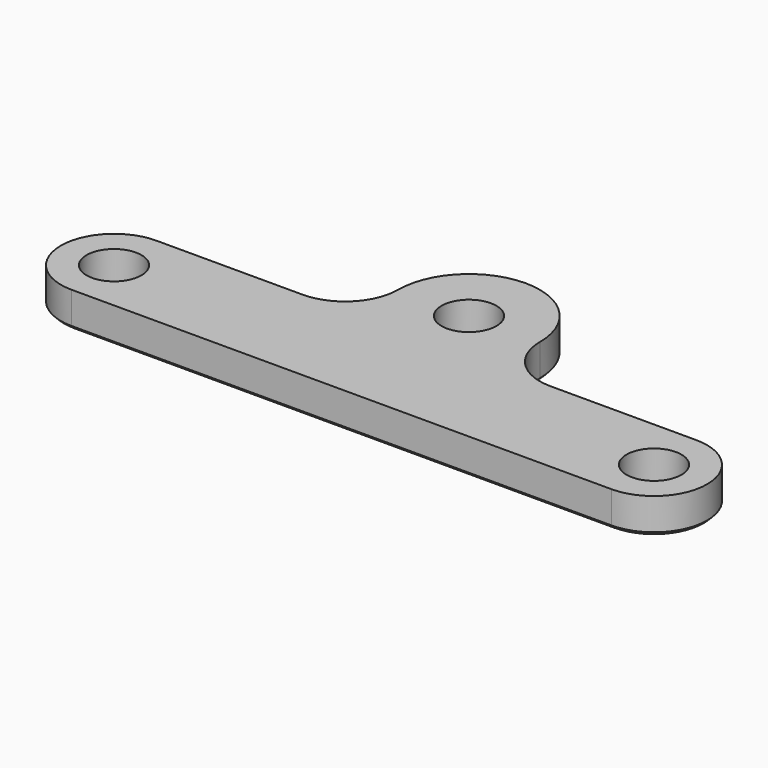
from build123d import *

# Parameters (mm, degrees)
F0_R     = 1.55
F1_DEPTH = 2
F2_R     = 2.99999
F3_SIZE  = 0.2


# Not quite as in the source:
# - a fillet or chamfer is up to 0.001 mm smaller than in the source, because OpenCascade refuses the exact size


with BuildPart() as f1:
    # F0 (on Top) → F1 (new body)
    with BuildSketch(Plane.XY):
        with BuildLine():
            ThreePointArc((-15.25, 3), (-18.25, 0), (-15.25, -3))
            Line((-15.25, -3), (15.25, -3))
            ThreePointArc((15.25, -3), (18.25, 0), (15.25, 3))
            Line((15.25, 3), (4, 3))
            Line((4, 3), (-4, 3))
            Line((-4, 3), (-15.25, 3))
        make_face()
        with Locations((-15.25, 0)):
            Circle(F0_R, mode=Mode.SUBTRACT)
        with Locations((15.25, 0)):
            Circle(F0_R, mode=Mode.SUBTRACT)
        with BuildLine():
            Line((-4, 6), (-4, 3))
            Line((-4, 3), (4, 3))
            Line((4, 3), (4, 6))
            ThreePointArc((4, 6), (0, 10), (-4, 6))
        make_face()
        with Locations((0, 6)):
            Circle(F0_R, mode=Mode.SUBTRACT)
    extrude(amount=F1_DEPTH)

    # F2 (radius 3 in the source; OpenCascade refuses exactly that, so slightly less here)
    f2_edges = [f1.edges().sort_by_distance(p)[0] for p in [
        (4, 3, 1),
        (-4, 3, 1),
    ]]
    fillet(f2_edges, radius=F2_R)

    # F3
    f3_edges = [f1.edges().sort_by_distance(p)[0] for p in [
        (11.124995, 3, 0),
        (4.878677, 3.878677, 0),
        (18.25, 0, 0),
        (4, 5.999995, 0),
        (0, -3, 0),
        (0, 10, 0),
        (-18.25, 0, 0),
        (-4, 5.999995, 0),
        (-11.124995, 3, 0),
        (-4.878677, 3.878677, 0),
        (-16.8, 0, 0),
        (13.7, 0, 0),
        (-1.55, 6, 0),
    ]]
    chamfer(f3_edges, length=F3_SIZE)


solid = f1.part
